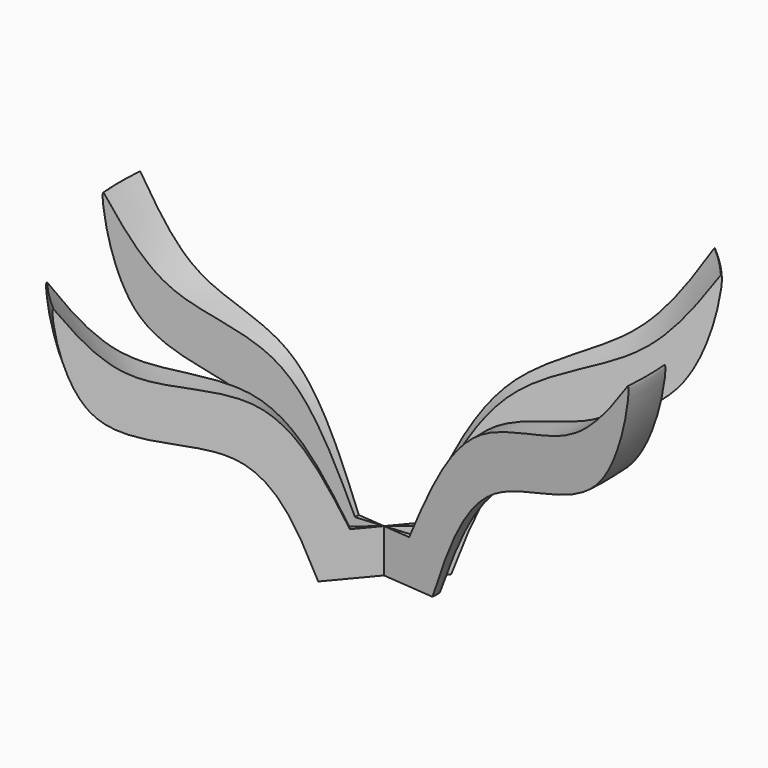
from build123d import *

# Parameters (mm, degrees)
F1_ANGLE_BACK = 5
F1_ANGLE      = 10
F3_COUNT      = 2


# Not quite as in the source:
# - a feature of the source that left no trace in its solid (it failed there, or was rolled back) is left out
# - a pattern or mirror of a feature is missing from the dataset's text; its kind, count and spacing are read off the source's solid


with BuildPart() as f1:
    # F0 (on Front) → F1 (revolve)
    with BuildSketch(Plane.XZ, mode=Mode.PRIVATE) as f1_sk:
        with BuildLine():
            add(Edge.make_bspline(
                [(-0.2524105464, 0), (-0.3307396385, 0.2256188139), (-0.4842284802, 0.6677274801), (-1.1998001381, 0.6252029855), (-1.2821282206, 1.2497196877), (-1.27, 1.2586820995), (-1.2686543401, 1.2596765041)],
                knots=[0, 0, 0, 0, 0.3404855991, 0.6671945103, 0.9630743035, 1, 1, 1, 1], degree=3))
            Line((-0.2524105464, 0), (0, 0))
            Line((0, 0), (0, 0.2095003059))
            Line((0, 0.2095003059), (-0.1308880734, 0.2095003059))
            add(Edge.make_bspline(
                [(-1.2686543401, 1.2596765041), (-1.1780005744, 1.133165691), (-0.9921915467, 0.8735596961), (-0.4159894857, 0.8570240231), (-0.230923084, 0.434631534), (-0.1308880734, 0.2095003059)],
                knots=[0, 0, 0, 0, 0.3061295799, 0.6268084555, 1, 1, 1, 1], degree=3))
        make_face()
    revolve(f1_sk.sketch.rotate(Axis((0, 0, 0.104750153), (0, 0, -1)), -F1_ANGLE_BACK), axis=Axis((0, 0, 0.104750153), (0, 0, -1)), revolution_arc=F1_ANGLE)

    # F1_copies: F1 across plane


with BuildPart() as f1_1:
    add(f1.part)
    add(f1.part.mirror(Plane(origin=(0, 0, 0), x_dir=(-0.3826834324, 0.9238795325, 0), z_dir=(0.9238795325, 0.3826834324, 0))))


with BuildPart() as f3_1:
    # F3: instance of F1
    add(f1_1.part.rotate(Axis((0, 0, 0.104750153), (0, 0, 1)), 1 * 360 / F3_COUNT))


solid = Compound([f1_1.part, f3_1.part])
